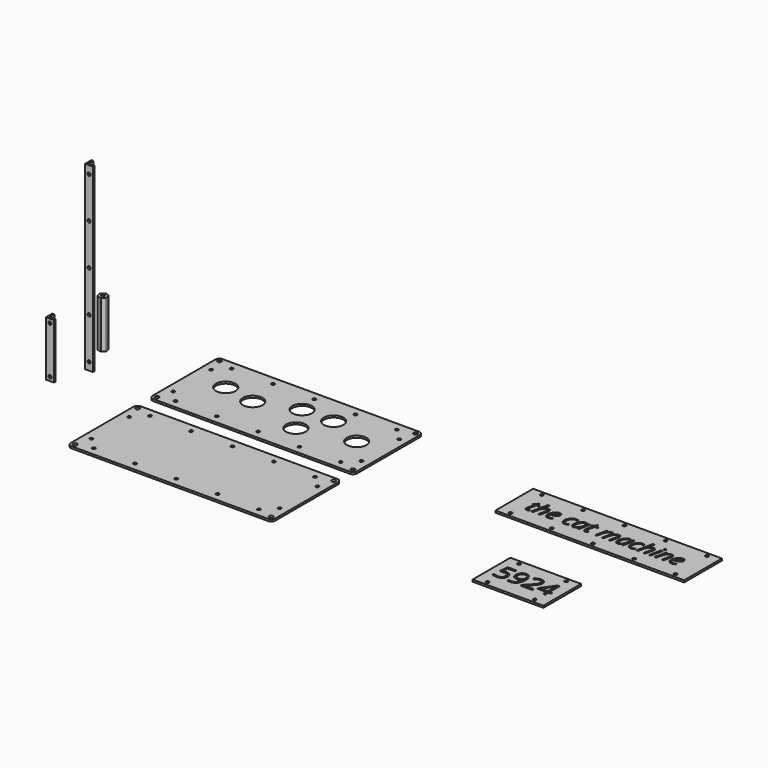
from build123d import *

# Parameters (mm, degrees)
F1_W             = 330.2
F1_H             = 139.7
F1_R             = 3.175
F1_R_2           = 2.54
F1_R_3           = 15.875
F2_DEPTH         = 3.175
F3_DEPTH         = 3.175
F1_W_2           = 304.8
F1_H_2           = 76.2
F4_DEPTH         = 3.175
F5_R             = 6.35
F5_2_R           = 6.35
F6_R             = 2.5527
F7_DEPTH         = 76.2
F9_DEPTH         = 292.1
F12_DEPTH        = 88.9
F15_D            = 5.08
F15_DEPTH        = 12.7
F15_TIP          = 1.5261859723
F15_ON_F11_D     = 5.08
F15_ON_F11_DEPTH = 12.7
F15_ON_F11_TIP   = 1.5261859723
F15_ON_F13_D     = 5.08
F15_ON_F13_DEPTH = 12.7
F15_ON_F13_TIP   = 1.5261859723
F15_ON_F14_D     = 5.08
F15_ON_F14_DEPTH = 12.7
F15_ON_F14_TIP   = 1.5261859723
F1_W_3           = 114.3
F16_DEPTH        = 3.175
F17_TEXT_SIZE    = 35.2777777778
F17_TEXT_SIZE_2  = 40.8820600973
F18_DEPTH        = 1.5875


# Not quite as in the source:
# - a length typed as a fraction of an inch, garbled in the dataset ("3 / 203.2 mm" for 3/8 in), is restored
# - Text() gives the source's letters only with a copy of the font that has no kerning and outlines rounded to 1/6400 em; it was checked with that copy


with BuildPart() as f2:
    # F1 (on Top) → F2 (new body)
    with BuildSketch(Plane.XY):
        with Locations((32.9742782729, 52.2314230949)):
            Rectangle(F1_W, F1_H)
        with Locations((-125.2550217271, -10.7478769051)):
            Circle(F1_R, mode=Mode.SUBTRACT)
        with Locations((-100.3757217271, -4.3978769051)):
            Circle(F1_R_2, mode=Mode.SUBTRACT)
        with Locations((-33.7007217271, -4.3978769051)):
            Circle(F1_R_2, mode=Mode.SUBTRACT)
        with Locations((32.9742782729, -4.3978769051)):
            Circle(F1_R_2, mode=Mode.SUBTRACT)
        with Locations((-118.9050217271, 14.1314230949)):
            Circle(F1_R_2, mode=Mode.SUBTRACT)
        with Locations((64.2035782729, 32.6607230949)):
            Circle(F1_R_3, mode=Mode.SUBTRACT)
        with Locations((99.6492782729, -4.3978769051)):
            Circle(F1_R_2, mode=Mode.SUBTRACT)
        with Locations((166.3242782729, -4.3978769051)):
            Circle(F1_R_2, mode=Mode.SUBTRACT)
        with Locations((191.2035782729, -10.7478769051)):
            Circle(F1_R, mode=Mode.SUBTRACT)
        with Locations((184.8535782729, 14.1314230949)):
            Circle(F1_R_2, mode=Mode.SUBTRACT)
        with Locations((-74.4550217271, 64.4107230949)):
            Circle(F1_R_3, mode=Mode.SUBTRACT)
        with Locations((-23.6550217271, 55.453312475)):
            Circle(F1_R_3, mode=Mode.SUBTRACT)
        with Locations((38.8035782729, 77.1107230949)):
            Circle(F1_R_3, mode=Mode.SUBTRACT)
        with Locations((-118.9050217271, 90.3314230949)):
            Circle(F1_R_2, mode=Mode.SUBTRACT)
        with Locations((-100.3757217271, 108.8607230949)):
            Circle(F1_R_2, mode=Mode.SUBTRACT)
        with Locations((-125.2550217271, 115.2107230949)):
            Circle(F1_R, mode=Mode.SUBTRACT)
        with Locations((-33.7007217271, 108.8607230949)):
            Circle(F1_R_2, mode=Mode.SUBTRACT)
        with Locations((32.9742782729, 108.8607230949)):
            Circle(F1_R_2, mode=Mode.SUBTRACT)
        with Locations((146.7535782729, 52.2314230949)):
            Circle(F1_R_3, mode=Mode.SUBTRACT)
        with Locations((89.6035782729, 77.1107230949)):
            Circle(F1_R_3, mode=Mode.SUBTRACT)
        with Locations((99.6492782729, 108.8607230949)):
            Circle(F1_R_2, mode=Mode.SUBTRACT)
        with Locations((166.3242782729, 108.8607230949)):
            Circle(F1_R_2, mode=Mode.SUBTRACT)
        with Locations((184.8535782729, 90.3314230949)):
            Circle(F1_R_2, mode=Mode.SUBTRACT)
        with Locations((191.2035782729, 115.2107230949)):
            Circle(F1_R, mode=Mode.SUBTRACT)
    extrude(amount=F2_DEPTH)

    # F5
    f5_edges = [f2.edges().sort_by_distance(p)[0] for p in [
        (-132.125722, -17.618577, 1.5875),
        (-132.125722, 122.081423, 1.5875),
        (198.074278, 122.081423, 1.5875),
        (198.074278, -17.618577, 1.5875),
    ]]
    fillet(f5_edges, radius=F5_R)


with BuildPart() as f3:
    # F1 (on Top) → F3 (new body)
    with BuildSketch(Plane.XY):
        with Locations((32.9742782729, -112.8685769051)):
            Rectangle(F1_W, F1_H)
        with Locations((-125.2550217271, -175.8478769051)):
            Circle(F1_R, mode=Mode.SUBTRACT)
        with Locations((-100.3757217271, -169.4978769051)):
            Circle(F1_R_2, mode=Mode.SUBTRACT)
        with Locations((-33.7007217271, -169.4978769051)):
            Circle(F1_R_2, mode=Mode.SUBTRACT)
        with Locations((-118.9050217271, -150.9685769051)):
            Circle(F1_R_2, mode=Mode.SUBTRACT)
        with Locations((32.9742782729, -169.4978769051)):
            Circle(F1_R_2, mode=Mode.SUBTRACT)
        with Locations((99.6492782729, -169.4978769051)):
            Circle(F1_R_2, mode=Mode.SUBTRACT)
        with Locations((166.3242782729, -169.4978769051)):
            Circle(F1_R_2, mode=Mode.SUBTRACT)
        with Locations((191.2035782729, -175.8478769051)):
            Circle(F1_R, mode=Mode.SUBTRACT)
        with Locations((184.8535782729, -150.9685769051)):
            Circle(F1_R_2, mode=Mode.SUBTRACT)
        with Locations((-118.9050217271, -74.7685769051)):
            Circle(F1_R_2, mode=Mode.SUBTRACT)
        with Locations((-125.2550217271, -49.8892769051)):
            Circle(F1_R, mode=Mode.SUBTRACT)
        with Locations((-100.3757217271, -56.2392769051)):
            Circle(F1_R_2, mode=Mode.SUBTRACT)
        with Locations((-33.7007217271, -56.2392769051)):
            Circle(F1_R_2, mode=Mode.SUBTRACT)
        with Locations((32.9742782729, -56.2392769051)):
            Circle(F1_R_2, mode=Mode.SUBTRACT)
        with Locations((184.8535782729, -74.7685769051)):
            Circle(F1_R_2, mode=Mode.SUBTRACT)
        with Locations((99.6492782729, -56.2392769051)):
            Circle(F1_R_2, mode=Mode.SUBTRACT)
        with Locations((166.3242782729, -56.2392769051)):
            Circle(F1_R_2, mode=Mode.SUBTRACT)
        with Locations((191.2035782729, -49.8892769051)):
            Circle(F1_R, mode=Mode.SUBTRACT)
    extrude(amount=F3_DEPTH)

    # F5#2
    f5_2_edges = [f3.edges().sort_by_distance(p)[0] for p in [
        (-132.125722, -43.018577, 1.5875),
        (-132.125722, -182.718577, 1.5875),
        (198.074278, -182.718577, 1.5875),
        (198.074278, -43.018577, 1.5875),
    ]]
    fillet(f5_2_edges, radius=F5_2_R)


with BuildPart() as f4:
    # F1 (on Top) → F4 (new body)
    with BuildSketch(Plane.XY):
        with Locations((553.6742782729, 52.2314230949)):
            Rectangle(F1_W_2, F1_H_2)
        with Locations((420.3242782729, 20.4814230949)):
            Circle(F1_R_2, mode=Mode.SUBTRACT)
        with Locations((486.9992782729, 20.4814230949)):
            Circle(F1_R_2, mode=Mode.SUBTRACT)
        with Locations((553.6742782729, 20.4814230949)):
            Circle(F1_R_2, mode=Mode.SUBTRACT)
        with Locations((620.3492782729, 20.4814230949)):
            Circle(F1_R_2, mode=Mode.SUBTRACT)
        with Locations((687.0242782729, 20.4814230949)):
            Circle(F1_R_2, mode=Mode.SUBTRACT)
        with Locations((420.3242782729, 83.9814230949)):
            Circle(F1_R_2, mode=Mode.SUBTRACT)
        with Locations((486.9992782729, 83.9814230949)):
            Circle(F1_R_2, mode=Mode.SUBTRACT)
        with Locations((553.6742782729, 83.9814230949)):
            Circle(F1_R_2, mode=Mode.SUBTRACT)
        with Locations((620.3492782729, 83.9814230949)):
            Circle(F1_R_2, mode=Mode.SUBTRACT)
        with Locations((687.0242782729, 83.9814230949)):
            Circle(F1_R_2, mode=Mode.SUBTRACT)
    extrude(amount=F4_DEPTH)


with BuildPart() as f7:
    # F6 (on Top) → F7 (new body)
    with BuildSketch(Plane.XY):
        with BuildLine():
            Line((-261.6749258704, 47.1374812706), (-257.748710844, 50.6189909326))
            ThreePointArc((-257.748710844, 50.6189909326), (-257.4067096677, 51.456596627), (-257.1777305195, 52.3318775268))
            Line((-257.1777305195, 52.3318775268), (-258.2296988172, 57.4728343113))
            ThreePointArc((-258.2296988172, 57.4728343113), (-258.7840860386, 58.1878188654), (-259.4276119592, 58.8237610745))
            Line((-259.4276119592, 58.8237610745), (-264.4057952832, 60.483208197))
            ThreePointArc((-264.4057952832, 60.483208197), (-265.3021836811, 60.3605870567), (-266.1746887498, 60.1212483661))
            Line((-266.1746887498, 60.1212483661), (-270.1009037762, 56.639738704))
            ThreePointArc((-270.1009037762, 56.639738704), (-270.4429049526, 55.8021330097), (-270.6718841007, 54.9268521099))
            Line((-270.6718841007, 54.9268521099), (-269.6199158031, 49.7858953253))
            ThreePointArc((-269.6199158031, 49.7858953253), (-269.0655285816, 49.0709107713), (-268.422002661, 48.4349685622))
            Line((-268.422002661, 48.4349685622), (-263.443819337, 46.7755214396))
            ThreePointArc((-263.443819337, 46.7755214396), (-262.5474309391, 46.8981425799), (-261.6749258704, 47.1374812706))
        make_face()
        with Locations((-263.9248073101, 53.6293648183)):
            Circle(F6_R, mode=Mode.SUBTRACT)
    extrude(amount=F7_DEPTH)


with BuildPart() as f9:
    # F8 (on Top) → F9 (new body)
    with BuildSketch(Plane.XY):
        Polygon((-244.3114764083, 9.6805094413), (-247.4864764083, 9.6805094413), (-247.4864764083, -3.0194905587), (-234.7864764083, -3.0194905587), (-234.7864764083, 0.1555094413), (-244.3114764083, 0.1555094413), align=None)
    extrude(amount=F9_DEPTH)

    # F15
    with Locations(Plane(origin=(-247.4864764083, 0, 0), x_dir=(0, -1, 0), z_dir=(-1, 0, 0))):
        with Locations((-3.3305094413, 279.4), (-3.3305094413, 212.725), (-3.3305094413, 146.05), (-3.3305094413, 79.375), (-3.3305094413, 12.7)):
            Hole(F15_D / 2, depth=F15_DEPTH)
            with Locations((0, 0, -(F15_DEPTH + F15_TIP / 2))):  # 118° drill point
                Cone(0, F15_D / 2, F15_TIP, mode=Mode.SUBTRACT)

    # F15 on F11
    with Locations(Plane.XZ.offset(3.0194905587)):
        with Locations((-241.1364764083, 279.4), (-241.1364764083, 212.725), (-241.1364764083, 146.05), (-241.1364764083, 79.375), (-241.1364764083, 12.7)):
            Hole(F15_ON_F11_D / 2, depth=F15_ON_F11_DEPTH)
            with Locations((0, 0, -(F15_ON_F11_DEPTH + F15_ON_F11_TIP / 2))):  # 118° drill point
                Cone(0, F15_ON_F11_D / 2, F15_ON_F11_TIP, mode=Mode.SUBTRACT)


with BuildPart() as f12:
    # F8 (on Top) → F12 (new body)
    with BuildSketch(Plane.XY):
        Polygon((-264.8357046604, -43.5430497944), (-268.0107046604, -43.5430497944), (-268.0107046604, -56.2430497944), (-255.3107046604, -56.2430497944), (-255.3107046604, -53.0680497944), (-264.8357046604, -53.0680497944), align=None)
    extrude(amount=F12_DEPTH)

    # F15 on F13
    with Locations(Plane(origin=(-268.0107046604, 0, 0), x_dir=(0, -1, 0), z_dir=(-1, 0, 0))):
        with Locations((49.8930497944, 82.55), (49.8930497944, 6.35)):
            Hole(F15_ON_F13_D / 2, depth=F15_ON_F13_DEPTH)
            with Locations((0, 0, -(F15_ON_F13_DEPTH + F15_ON_F13_TIP / 2))):  # 118° drill point
                Cone(0, F15_ON_F13_D / 2, F15_ON_F13_TIP, mode=Mode.SUBTRACT)

    # F15 on F14
    with Locations(Plane.XZ.offset(56.2430497944)):
        with Locations((-261.6607046604, 82.55), (-261.6607046604, 6.35)):
            Hole(F15_ON_F14_D / 2, depth=F15_ON_F14_DEPTH)
            with Locations((0, 0, -(F15_ON_F14_DEPTH + F15_ON_F14_TIP / 2))):  # 118° drill point
                Cone(0, F15_ON_F14_D / 2, F15_ON_F14_TIP, mode=Mode.SUBTRACT)


with BuildPart() as f16:
    # F1 (on Top) → F16 (new body)
    with BuildSketch(Plane.XY):
        with Locations((553.6742782729, -112.8685769051)):
            Rectangle(F1_W_3, F1_H_2)
        with Locations((515.5742782729, -144.6185769051)):
            Circle(F1_R_2, mode=Mode.SUBTRACT)
        with Locations((591.7742782729, -144.6185769051)):
            Circle(F1_R_2, mode=Mode.SUBTRACT)
        with Locations((515.5742782729, -81.1185769051)):
            Circle(F1_R_2, mode=Mode.SUBTRACT)
        with Locations((591.7742782729, -81.1185769051)):
            Circle(F1_R_2, mode=Mode.SUBTRACT)
    extrude(amount=F16_DEPTH)


with BuildPart() as f18_tool:
    # F17 (on face) → F18 (new body)
    with BuildSketch(Plane.XY.offset(3.175)):
        with Locations((425.5461806936, 40.1633914748)):
            Text('the cat machine', F17_TEXT_SIZE, font='Open Sans', font_style=FontStyle.ITALIC, text_align=(TextAlign.LEFT, TextAlign.BOTTOM))
        with Locations((505.4255723953, -126.3163462281)):
            Text('5924', F17_TEXT_SIZE_2, font='Open Sans', text_align=(TextAlign.LEFT, TextAlign.BOTTOM))
    extrude(amount=-F18_DEPTH)


with BuildPart() as f4_1:
    add(f4.part)

    # F18: cut by f18_tool
    add(f18_tool.part, mode=Mode.SUBTRACT)


with BuildPart() as f16_1:
    add(f16.part)

    # F18: cut by f18_tool
    add(f18_tool.part, mode=Mode.SUBTRACT)


solid = Compound([f2.part, f3.part, f7.part, f9.part, f12.part, f4_1.part, f16_1.part])
